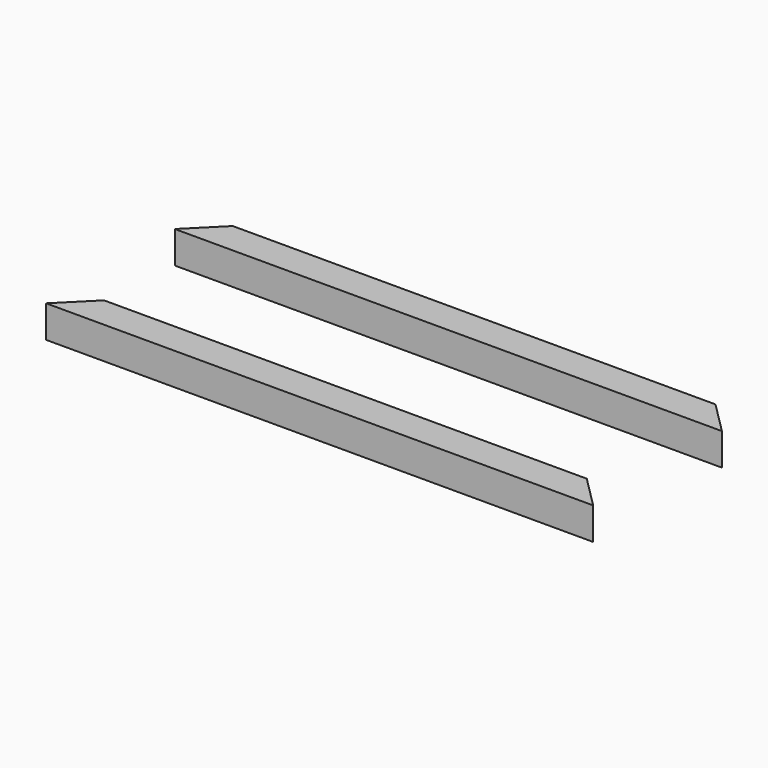
from build123d import *

# Parameters (mm, degrees)
F0_W        = 863.6
F0_H        = 50.8
F1_DEPTH    = 50.8
F2_W        = 44.45
F2_H        = 44.45
F3_DEPTH    = 863.601
F4_T1_DEPTH = 312.0829915773


# Not quite as in the source:
# - a fillet or chamfer that OpenCascade refuses, or shapes differently, is made with other operations: its cross-section is extruded or revolved along the edge and cut away or added


with BuildPart() as f1:
    # F0 (on Front) → F1 (new body)
    with BuildSketch(Plane.XZ):
        Rectangle(F0_W, F0_H)
    extrude(amount=F1_DEPTH)

    # F2 (on face) → F3 (cut, through all)
    with BuildSketch(Plane(origin=(-431.8, 0, 0), x_dir=(0, -1, 0), z_dir=(-1, 0, 0))):
        with Locations((25.4, 0)):
            Rectangle(F2_W, F2_H)
    extrude(amount=-F3_DEPTH, mode=Mode.SUBTRACT)

    # F4: chamfer of 50.8 on 2 edges, made by hand

    # F4_s2 → F4_t1 (cut)
    with BuildSketch(Plane.XY.offset(-156.0414957887)):
        Polygon((431.8, -50.8), (381, 0), (431.8, 0), align=None)
        Polygon((-381, 0), (-431.8, -50.8), (-431.8, 0), align=None)
    extrude(amount=F4_T1_DEPTH, mode=Mode.SUBTRACT)


with BuildPart() as f5_1:
    # F5: copy of F1
    add(f1.part.moved(Location((0, 254, 0))))


solid = Compound([f1.part, f5_1.part])
